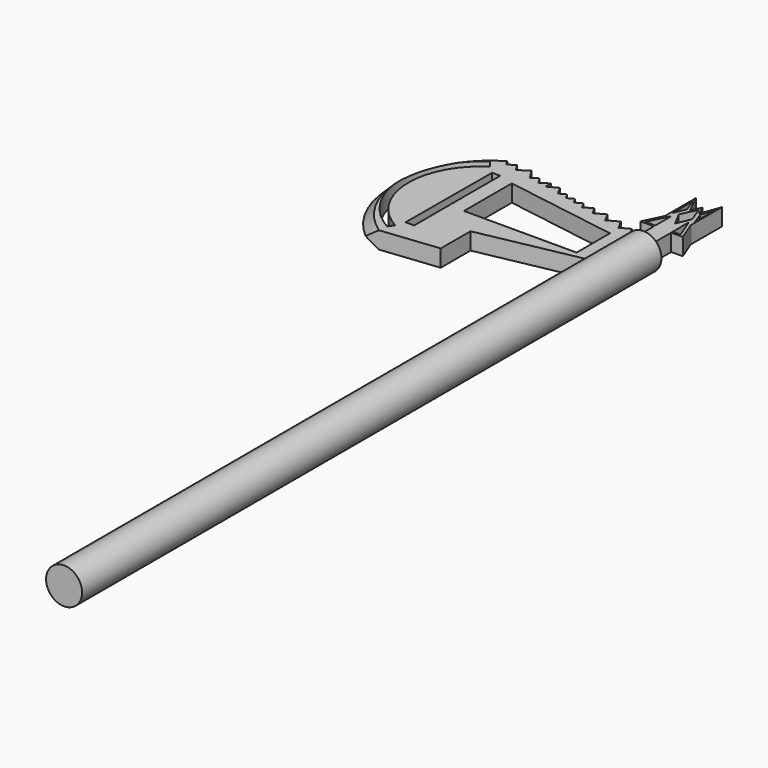
from build123d import *

# Parameters (mm, degrees)
F0_R          = 5.373622476
F1_DEPTH      = 215.88753
F3_DEPTH      = 2.54
F3_DEPTH_BACK = 2.54
F4_T2_ANGLE   = 126.5345537541
F4_T4_ANGLE   = 126.5345537541


# Not quite as in the source:
# - a fillet or chamfer that OpenCascade refuses, or shapes differently, is made with other operations: its cross-section is extruded or revolved along the edge and cut away or added


with BuildPart() as f1:
    # F0 (on Front) → F1 (new body)
    with BuildSketch(Plane.XZ):
        Circle(F0_R)
    extrude(amount=F1_DEPTH)

    # F2 (on Top) → F3 (join, two sides)
    with BuildSketch(Plane.XY) as f3_sk:
        Polygon((-8.9527533501, 1.9022722074), (-4.8790749139, 1.0367010286), (-6.158160232, 3.4090294491), align=None)
        Polygon((-13.7193289536, 2.9150694934), (-8.9527533501, 1.9022722074), (-10.4493999233, 4.6781129985), align=None)
        Polygon((-18.2748671635, 3.8830257621), (-13.7193289536, 2.9150694934), (-15.1497123605, 5.5680115299), align=None)
        Polygon((-22.0207331241, 4.6789436692), (-18.2748671635, 3.8830257621), (-19.4510233645, 6.0644508345), align=None)
        Polygon((-25.0378297706, 5.3200133908), (-22.0207331241, 4.6789436692), (-22.9680646536, 6.4359660347), align=None)
        Polygon((-27.890320124, 5.9261077295), (-25.0378297706, 5.3200133908), (-25.9334769328, 6.9811764013), align=None)
        Polygon((-28.7897214748, 7.5942336596), (-30.7547669567, 6.5347425691), (-27.890320124, 5.9261077295), align=None)
        Polygon((-32.1493126453, 9.1212161407), (-35.1961678702, 7.4784470575), (-30.7547669567, 6.5347425691), align=None)
        Polygon((-35.1961678702, 9.5456602661), (-37.6418792182, 7.9981093941), (-35.1961678702, 7.4784470575), align=None)
        Polygon((-38.8515780683, 9.9098877134), (-40.8092972733, 8.6711192604), (-37.6418792182, 7.9981093941), align=None)
        Polygon((-42.7175686579, 11.6869044373), (-45.8058244977, 9.7327764402), (-40.8092972733, 8.6711192604), align=None)
        Polygon((-47.1321087681, 11.8288034913), (-49.2785042842, 10.4706480183), (-45.8058244977, 9.7327764402), align=None)
        Polygon((-50.8480016213, 12.9510430201), (-53.3880016213, 11.343829962), (-49.2785042842, 10.4706480183), align=None)
        Polygon((-2.9497377109, 0), (0, 0), (-2.9497377109, 0.6267573614), align=None)
        Polygon((1.198072837, 19.0015498009), (3.3619815949, 13.447928708), (3.3619815949, 25.0585451722), align=None)
        Polygon((3.0523012392, 22.8999685496), (3.0523012392, 15.3504825952), (1.7903243424, 18.9260840416), align=None, mode=Mode.SUBTRACT)
        Polygon((-4.2252911557, 24.8437412083), (-4.2252911557, 13.2858192763), (-1.4181542095, 19.1259601465), align=None)
        Polygon((-3.7408936769, 22.9805186391), (-2.2895061411, 19.10783723), (-3.7408936769, 15.6503133476), align=None, mode=Mode.SUBTRACT)
        Polygon((-2.9497377109, 0.6267573614), (0, 0), (2.1719516162, 0), (2.1719516162, 7.62), (5.6152132711, 7.6650624399), (3.3619815949, 13.447928708), (1.198072837, 19.0015498009), (0, 22.0763756473), (-1.4181542095, 19.1259601465), (-4.2252911557, 13.2858192763), (-6.9486382417, 7.62), (-2.9497377109, 7.62), align=None)
        Polygon((-2.9854448512, 13.0213079974), (-2.9854448512, 8.1413947046), (-5.9038246982, 8.1413947046), (-2.9854448512, 14.2129721679), align=None, mode=Mode.SUBTRACT)
        Polygon((2.1099960018, 14.3143812405), (4.47795121, 8.2370797172), (2.1719516162, 8.2069007827), (2.1089701391, 13.0193722181), align=None, mode=Mode.SUBTRACT)
        Polygon((-2.2104110103, 15.9188192338), (0, 20.6176694483), (1.7634738469, 15.9993711859), (0, 11.8375318125), align=None, mode=Mode.SUBTRACT)
        with BuildLine():
            Line((-34.7528146772, -32.0806060351), (-34.7528146772, -20.9908965406))
            Line((-34.7528146772, -20.9908965406), (0, -14.0988837661))
            Line((0, -14.0988837661), (0, 0))
            Line((0, 0), (-2.9497377109, 0))
            Line((-2.9497377109, 0), (-2.9497377109, 0.6267573614))
            Line((-2.9497377109, 0.6267573614), (-4.8790749139, 1.0367010286))
            Line((-4.8790749139, 1.0367010286), (-8.9527533501, 1.9022722074))
            Line((-8.9527533501, 1.9022722074), (-13.7193289536, 2.9150694934))
            Line((-13.7193289536, 2.9150694934), (-18.2748671635, 3.8830257621))
            Line((-18.2748671635, 3.8830257621), (-22.0207331241, 4.6789436692))
            Line((-22.0207331241, 4.6789436692), (-25.0378297706, 5.3200133908))
            Line((-25.0378297706, 5.3200133908), (-27.890320124, 5.9261077295))
            Line((-27.890320124, 5.9261077295), (-30.7547669567, 6.5347425691))
            Line((-30.7547669567, 6.5347425691), (-35.1961678702, 7.4784470575))
            Line((-35.1961678702, 7.4784470575), (-37.6418792182, 7.9981093941))
            Line((-37.6418792182, 7.9981093941), (-40.8092972733, 8.6711192604))
            Line((-40.8092972733, 8.6711192604), (-45.8058244977, 9.7327764402))
            Line((-45.8058244977, 9.7327764402), (-49.2785042842, 10.4706480183))
            Line((-49.2785042842, 10.4706480183), (-53.3880016213, 11.343829962))
            Line((-53.3880016213, 11.343829962), (-54.9966600991, 11.6856361297))
            ThreePointArc((-54.9966600991, 11.6856361297), (-66.0747003656, -11.2262862037), (-55.3715413676, -34.3157112426))
            Line((-55.3715413676, -34.3157112426), (-34.7528146772, -32.0806060351))
        make_face()
        with BuildLine():
            ThreePointArc((-51.421571523, -31.2265530229), (-63.6234506771, -11.4887260787), (-53.1807132065, 9.2336507514))
            Line((-53.1807132065, 9.2336507514), (-51.5400195681, 7.2946498786))
            ThreePointArc((-51.5400195681, 7.2946498786), (-61.3618234836, -11.493283063), (-50.339024514, -29.6027325094))
            Line((-50.339024514, -29.6027325094), (-51.421571523, -31.2265530229))
        make_face(mode=Mode.SUBTRACT)
        Polygon((-49.3917986751, -26.8963649869), (-49.256477505, 5.174099002), (-46.8207485974, 5.174099002), (-46.8207485974, -26.8963649869), align=None, mode=Mode.SUBTRACT)
        Polygon((-42.3252023757, 3.8717763964), (-8.7594440334, -1.5370512847), (-8.7594440334, -13.9601901174), (-42.3252023757, -13.9601901174), (-42.3252023757, -1.5370512847), align=None, mode=Mode.SUBTRACT)
    extrude(amount=F3_DEPTH)
    extrude(f3_sk.sketch, amount=-F3_DEPTH_BACK)

    # F4: chamfer of 2.54 on 2 edges, made by hand

    # F4_s1 → F4_t2 (revolve, cut)
    with BuildSketch(Plane(origin=(-33.7752745406, -16.6677099753, 0), x_dir=(0, 0, 1), z_dir=(0.8967506648, 0.4425361512, 0))):
        Polygon((0, -35.5324348562), (2.54, -32.9924348562), (2.54, -35.5324348562), align=None)
    revolve(axis=Axis((-36.340977144, -11.4685968428, 2.54), (0, 0, 1)), revolution_arc=F4_T2_ANGLE, mode=Mode.SUBTRACT)

    # F4_s3 → F4_t4 (revolve, cut)
    with BuildSketch(Plane(origin=(-33.7752745406, -16.6677099753, 0), x_dir=(0, 0, 1), z_dir=(0.8967506648, 0.4425361512, 0))):
        Polygon((-2.54, -32.9924348562), (0, -35.5324348562), (-2.54, -35.5324348562), align=None)
    revolve(axis=Axis((-36.340977144, -11.4685968428, -2.54), (0, 0, 1)), revolution_arc=F4_T4_ANGLE, mode=Mode.SUBTRACT)


solid = f1.part
